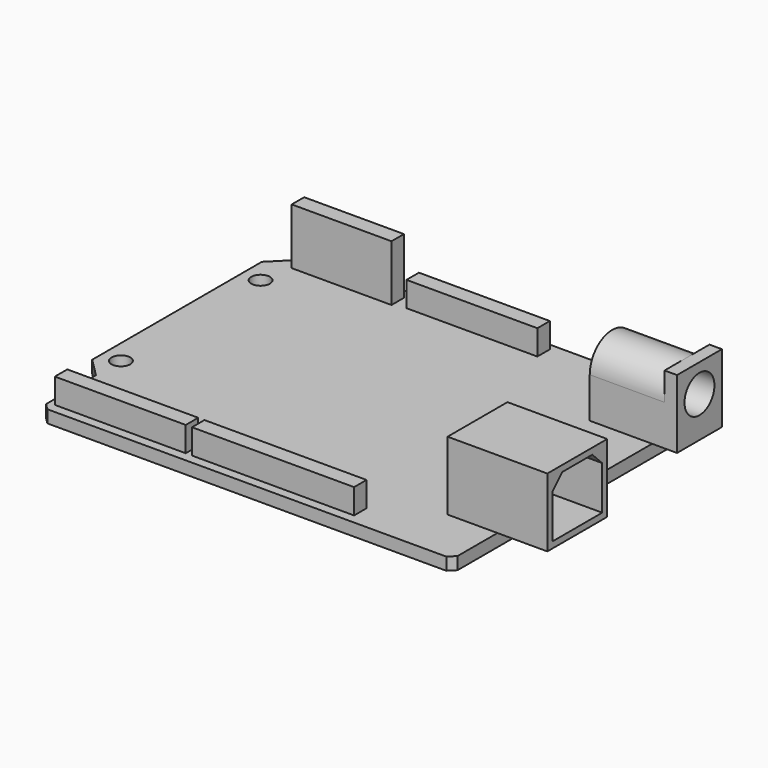
from build123d import *

# Parameters (mm, degrees)
F1_DEPTH  = 2
F2_W      = 16
F2_H      = 12
F3_DEPTH  = 11
F4_W      = 14
F4_H      = 9
F5_DEPTH  = 11
F6_W      = 16
F6_H      = 2.5
F7_DEPTH  = 9
F8_W      = 21
F8_H      = 2.5
F9_DEPTH  = 4
F10_W     = 21
F10_H     = 2.5
F10_W_2   = 26
F11_DEPTH = 4
F13_DEPTH = 12
F14_R     = 3
F15_DEPTH = 12
F17_DEPTH = 12
F18_SIZE2 = 2.99999
F18_SIZE  = 2.99999
F19_SIZE2 = 1
F19_SIZE  = 1
F20_R     = 1.5
F21_DEPTH = 2


# Not quite as in the source:
# - a fillet or chamfer is up to 0.001 mm smaller than in the source, because OpenCascade refuses the exact size


with BuildPart() as f1:
    # F0 (on Top) → F1 (new body)
    with BuildSketch(Plane.XY):
        Polygon((3, 11), (3, 0), (69, 0), (69, 53), (3, 53), (3, 51), (0, 51), (0, 11), align=None)
    extrude(amount=F1_DEPTH)

    # F2 (on face) → F3 (join)
    with BuildSketch(Plane.XY.offset(2)):
        with Locations((69, 15)):
            Rectangle(F2_W, F2_H)
    extrude(amount=F3_DEPTH)

    # F4 (on face) → F5 (join)
    with BuildSketch(Plane.XY.offset(2)):
        with Locations((66, 44.5)):
            Rectangle(F4_W, F4_H)
    extrude(amount=F5_DEPTH)

    # F6 (on face) → F7 (join)
    with BuildSketch(Plane.XY.offset(2)):
        with Locations((12, 50.25)):
            Rectangle(F6_W, F6_H)
    extrude(amount=F7_DEPTH)

    # F8 (on face) → F9 (join)
    with BuildSketch(Plane.XY.offset(2)):
        with Locations((32.5, 50.75)):
            Rectangle(F8_W, F8_H)
    extrude(amount=F9_DEPTH)

    # F10 (on face) → F11 (join)
    with BuildSketch(Plane.XY.offset(2)):
        with Locations((14.5, 2.75)):
            Rectangle(F10_W, F10_H)
        with Locations((39, 2.75)):
            Rectangle(F10_W_2, F10_H)
    extrude(amount=F11_DEPTH)

    # F12 (on face) → F13 (cut)
    with BuildSketch(Plane(origin=(59, 0, 0), x_dir=(0, -1, 0), z_dir=(-1, 0, 0))):
        with BuildLine():
            ThreePointArc((-49, 8.5), (-44.5, 13), (-40, 8.5))
            Line((-40, 8.5), (-38.6329554021, 9.580289945))
            Line((-38.6329554021, 9.580289945), (-38.187738508, 14.0570942312))
            Line((-38.187738508, 14.0570942312), (-42.2688946128, 14.7991068661))
            Line((-42.2688946128, 14.7991068661), (-51.2474328279, 13.8839585707))
            Line((-51.2474328279, 13.8839585707), (-49, 8.5))
        make_face()
        Polygon((-40, 13), (-40, 8.5), (-38.6329554021, 9.580289945), (-38.187738508, 14.0570942312), (-42.2688946128, 14.7991068661), (-51.2474328279, 13.8839585707), (-49, 8.5), (-49, 13), (-44.5, 13), align=None)
    extrude(amount=-F13_DEPTH, mode=Mode.SUBTRACT)

    # F14 (on face) → F15 (cut)
    with BuildSketch(Plane.YZ.offset(73)):
        with Locations((44.5, 8.5)):
            Circle(F14_R)
    extrude(amount=-F15_DEPTH, mode=Mode.SUBTRACT)

    # F16 (on face) → F17 (cut)
    with BuildSketch(Plane.YZ.offset(77)):
        Polygon((18, 12), (12, 12), (10, 10), (10, 3), (20, 3), (20, 10), align=None)
    extrude(amount=-F17_DEPTH, mode=Mode.SUBTRACT)

    # F18 (size 3 and 3 in the source; OpenCascade refuses exactly that, so slightly less here)
    f18_edges = [f1.edges().sort_by_distance(p)[0] for p in [
        (0, 51, 1),
        (0, 11, 1),
    ]]
    chamfer(f18_edges, length=F18_SIZE, length2=F18_SIZE2)

    # F19
    f19_edges = [f1.edges().sort_by_distance(p)[0] for p in [
        (3, 0, 1),
        (69, 0, 1),
        (69, 53, 1),
        (3, 53, 1),
    ]]
    chamfer(f19_edges, length=F19_SIZE, length2=F19_SIZE2)

    # F20 (on face) → F21 (cut)
    with BuildSketch(Plane.XY.offset(2)):
        with Locations((3, 16)):
            Circle(F20_R)
        with Locations((3, 44)):
            Circle(F20_R)
    extrude(amount=-F21_DEPTH, mode=Mode.SUBTRACT)


solid = f1.part
